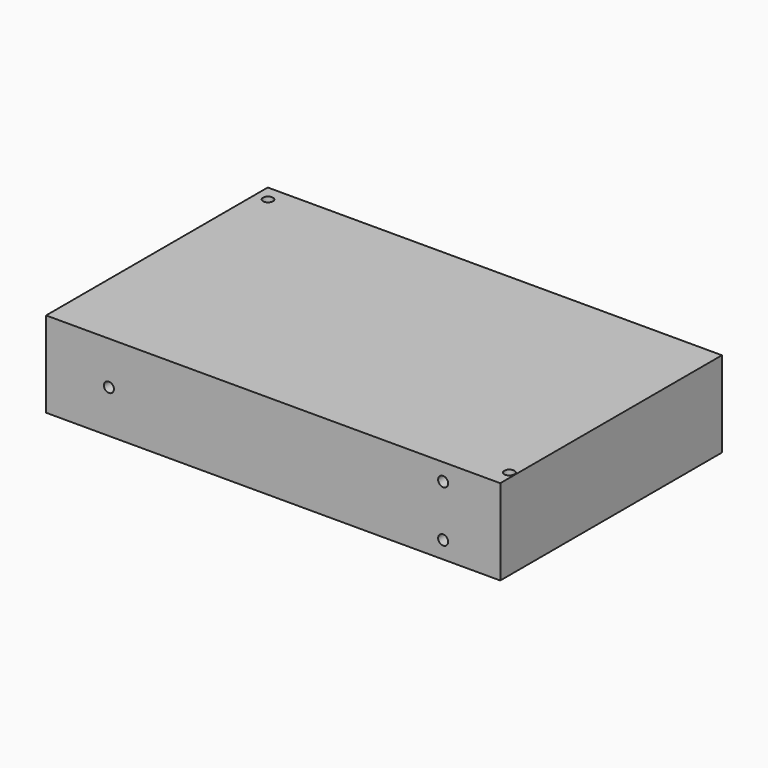
from build123d import *

# Parameters (mm, degrees)
F0_W     = 159
F0_H     = 97
F0_R     = 1.75
F1_DEPTH = 30
F2_R     = 1.75
F3_DEPTH = 25


# Not quite as in the source:
# - a pattern or mirror of a feature is missing from the dataset's text; its kind, count and spacing are read off the source's solid


with BuildPart() as f1:
    # F0 (on Top) → F1 (new body)
    with BuildSketch(Plane.XY):
        with Locations((36.3976350129, 66.932474792)):
            Rectangle(F0_W, F0_H)
        with Locations((113.8976350129, 24.932474792)):
            Circle(F0_R, mode=Mode.SUBTRACT)
        with Locations((-38.6023649871, 109.932474792)):
            Circle(F0_R, mode=Mode.SUBTRACT)
    extrude(amount=F1_DEPTH)

    # F2 (on face) → F3 (cut)
    with BuildSketch(Plane.XZ.offset(-18.432474792)):
        with Locations((-21.1023649871, 15)):
            Circle(F2_R)
        with Locations((95.8976350129, 24)):
            Circle(F2_R)
        with Locations((95.8976350129, 6)):
            Circle(F2_R)
    f3 = extrude(amount=-F3_DEPTH, mode=Mode.SUBTRACT)

    # F3_copies: F3 across plane
    add(f3.mirror(Plane.ZX.offset(66.932475)), mode=Mode.SUBTRACT)


solid = f1.part
